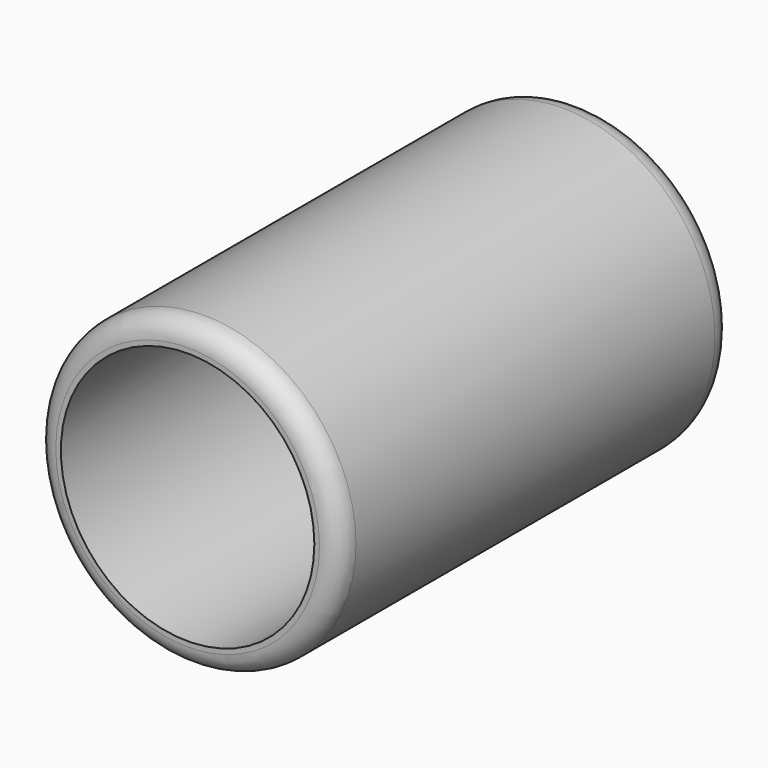
from build123d import *

# Parameters (mm, degrees)
F0_R     = 38.1
F0_R_2   = 31.75
F1_DEPTH = 123.825
F2_DEPTH = 15.24
F3_R     = 6.34999
F4_R     = 5.08


# Not quite as in the source:
# - a fillet or chamfer is up to 0.001 mm smaller than in the source, because OpenCascade refuses the exact size


with BuildPart() as f1:
    # F0 (on Front) → F1 (new body)
    with BuildSketch(Plane.XZ):
        Circle(F0_R)
        Circle(F0_R_2, mode=Mode.SUBTRACT)
    extrude(amount=F1_DEPTH)

    # F3 (radius 6.35 in the source; OpenCascade refuses exactly that, so slightly less here)
    f3_edges = [f1.edges().sort_by_distance(p)[0] for p in [
        (-38.1, 0, 0),
    ]]
    fillet(f3_edges, radius=F3_R)

    # F4
    f4_edges = [f1.edges().sort_by_distance(p)[0] for p in [
        (-38.1, -123.825, 0),
    ]]
    fillet(f4_edges, radius=F4_R)


with BuildPart() as f2:
    # F0 (on Front) → F2 (new body)
    with BuildSketch(Plane.XZ):
        Circle(F0_R_2)
    extrude(amount=F2_DEPTH)


solid = Compound([f1.part, f2.part])
